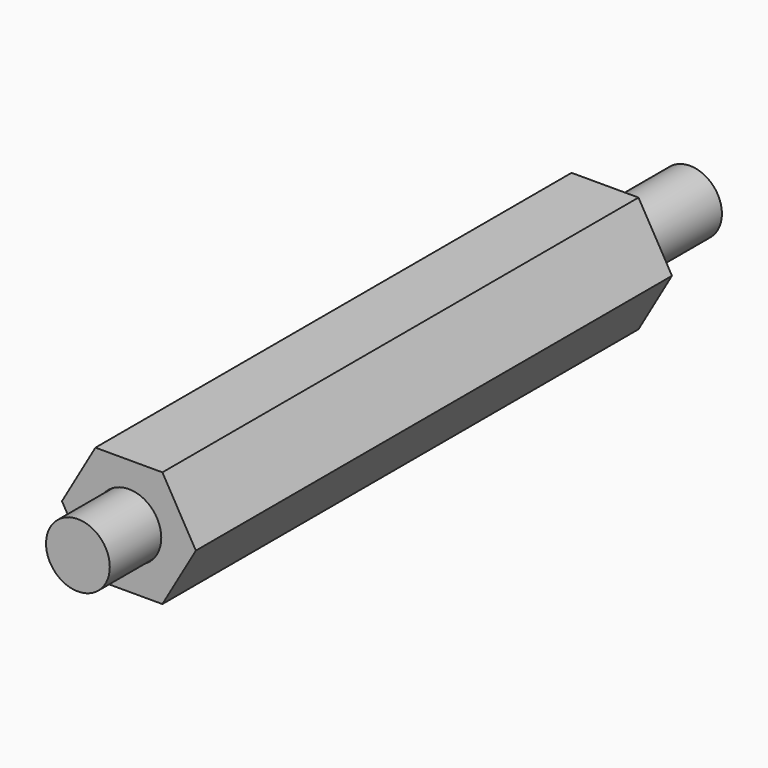
from build123d import *

# Parameters (mm, degrees)
F0_R     = 1.5223329882
F1_DEPTH = 28
F0_R_2   = 1.5
F2_DEPTH = 5
F3_DEPTH = 3


with BuildPart() as f1:
    # F0 (on Front) → F1 (new body)
    with BuildSketch(Plane.XZ):
        Polygon((-1.575, -2.7279800219), (1.575, -2.7279800219), (3.15, 0), (1.575, 2.7279800219), (-1.575, 2.7279800219), (-3.15, 0), align=None)
        Circle(F0_R, mode=Mode.SUBTRACT)
    extrude(amount=F1_DEPTH)


with BuildPart() as f1b:
    # F0 (on Front) → F1, piece 2 (new body)
    with BuildSketch(Plane.XZ):
        Circle(F0_R_2)
    extrude(amount=F1_DEPTH)

    # F3 (add): a face of the model
    f3_faces = [f1b.faces().sort_by_distance(p)[0] for p in [
        (0, -28, 0),
    ]]
    extrude(f3_faces, amount=F3_DEPTH)


with BuildPart() as f2:
    # F0 (on Front) → F2 (new body)
    with BuildSketch(Plane.XZ):
        Circle(F0_R_2)
    extrude(amount=-F2_DEPTH)


solid = Compound([f1.part, f1b.part, f2.part])
